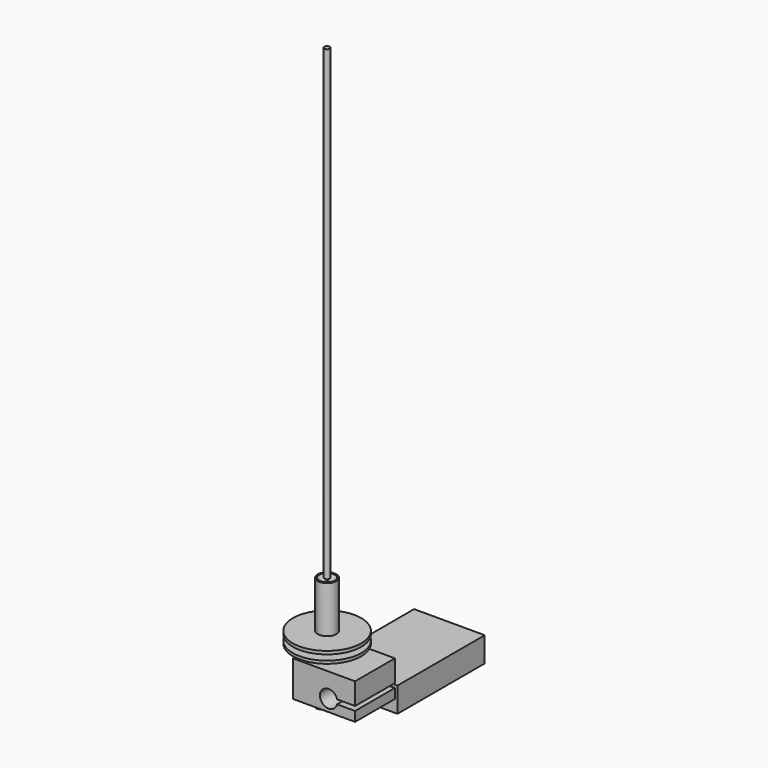
from build123d import *

# Parameters (mm, degrees)
F0_R      = 11
F1_DEPTH  = 1
F2_R      = 7
F3_DEPTH  = 1.76
F4_R      = 11
F5_DEPTH  = 0.9
F6_R      = 2
F7_DEPTH  = 2.4
F8_W      = 20
F8_H      = 16
F9_DEPTH  = 11.5
F10_R     = 2.8
F11_DEPTH = 19.001
F12_W     = 16
F12_H     = 1.4
F13_DEPTH = 5.7899116577
F15_DEPTH = 3
F16_R     = 2.25
F17_DEPTH = 2
F19_R     = 3
F20_DEPTH = 15
F21_R     = 0.2
F22_DEPTH = 37.561
F23_R     = 1
F24_DEPTH = 15.001
F25_SIZE  = 1.5
F27_W     = 22.7133790031
F27_H     = 35.0576061755
F28_DEPTH = 8
F30_R     = 0.875
F31_DEPTH = 150


# Not quite as in the source:
# - a fillet or chamfer that OpenCascade refuses, or shapes differently, is made with other operations: its cross-section is extruded or revolved along the edge and cut away or added


with BuildPart() as f1:
    # F0 (on Top) → F1 (new body)
    with BuildSketch(Plane.XY):
        Circle(F0_R)
    extrude(amount=-F1_DEPTH)

    # F2 (on face) → F3 (join)
    with BuildSketch(Plane(origin=(0, 0, -1), x_dir=(1, 0, 0), z_dir=(0, 0, -1))):
        Circle(F2_R)
    extrude(amount=F3_DEPTH)

    # F4 (on face) → F5 (join)
    with BuildSketch(Plane(origin=(0, 0, -2.76), x_dir=(1, 0, 0), z_dir=(0, 0, -1))):
        Circle(F4_R)
    extrude(amount=F5_DEPTH)

    # F6 (on face) → F7 (join)
    with BuildSketch(Plane(origin=(0, 0, -3.66), x_dir=(1, 0, 0), z_dir=(0, 0, -1))):
        Circle(F6_R)
    extrude(amount=F7_DEPTH)

    # F8 (on face) → F9 (join)
    with BuildSketch(Plane(origin=(0, 0, -6.06), x_dir=(1, 0, 0), z_dir=(0, 0, -1))):
        with Locations((5.4, 0)):
            Rectangle(F8_W, F8_H)
    extrude(amount=F9_DEPTH)

    # F10 (on face) → F11 (cut, through all)
    with BuildSketch(Plane.XZ.offset(8)):
        with Locations((6.9, -13.76)):
            Circle(F10_R)
    extrude(amount=-F11_DEPTH, mode=Mode.SUBTRACT)

    # F12 (on face) → F13 (cut, through all)
    with BuildSketch(Plane.YZ.offset(15.4)):
        with Locations((0, -13.76)):
            Rectangle(F12_W, F12_H)
    extrude(amount=-F13_DEPTH, mode=Mode.SUBTRACT)

    # F14 (on face) → F15 (join)
    with BuildSketch(Plane(origin=(0, 0, -17.56), x_dir=(1, 0, 0), z_dir=(0, 0, -1))):
        Polygon((0.0435586886, -4.0414518843), (3.5217793443, -1.9830030113), (3.4782206557, 2.058448873), (-0.0435586886, 4.0414518843), (-3.5217793443, 1.9830030113), (-3.4782206557, -2.058448873), align=None)
    extrude(amount=F15_DEPTH)

    # F16 (on face) → F17 (join)
    with BuildSketch(Plane(origin=(0, 0, -20.56), x_dir=(1, 0, 0), z_dir=(0, 0, -1))):
        Circle(F16_R)
    extrude(amount=F17_DEPTH)

    # F18: chamfer of 1.8 x 2.2 on 1 edges, made by hand


with BuildPart() as f18_tool2:
    # F18_s3 → F18_t4 (revolve)
    with BuildSketch(Plane.XZ):
        Polygon((2.25, -20.36), (0.45, -22.56), (2.25, -22.56), align=None)
    revolve(axis=Axis((0, 0, -22.56), (0, 0, -1)))

    split(bisect_by=Plane.XY.offset(-20.56), keep=Keep.BOTTOM)


with BuildPart() as f1_1:
    add(f1.part)

    # F18_t1: cut F18_tool2
    add(f18_tool2.part, mode=Mode.SUBTRACT)

    # F19 (on face) → F20 (join)
    with BuildSketch(Plane.XY):
        Circle(F19_R)
    extrude(amount=F20_DEPTH)

    # F21 (on face) → F22 (cut, through all)
    with BuildSketch(Plane(origin=(0, 0, -22.56), x_dir=(1, 0, 0), z_dir=(0, 0, -1))):
        Circle(F21_R)
    extrude(amount=-F22_DEPTH, mode=Mode.SUBTRACT)

    # F23 (on face) → F24 (cut, through all)
    with BuildSketch(Plane.XY):
        Circle(F23_R)
    extrude(amount=F24_DEPTH, mode=Mode.SUBTRACT)

    # F25
    f25_edges = [f1_1.edges().sort_by_distance(p)[0] for p in [
        (-1, 0, 15),
    ]]
    chamfer(f25_edges, length=F25_SIZE)


with BuildPart() as f28:
    # F27 (on offset) → F28 (new body)
    with BuildSketch(Plane.XY.offset(-22.6)):
        with Locations((3.563052509, 27.1755484864)):
            Rectangle(F27_W, F27_H)
    extrude(amount=F28_DEPTH)


with BuildPart() as f31:
    # F30 (on offset) → F31 (new body)
    with BuildSketch(Plane.XY.offset(15)):
        Circle(F30_R)
    extrude(amount=F31_DEPTH)


solid = Compound([f1_1.part, f28.part, f31.part])
